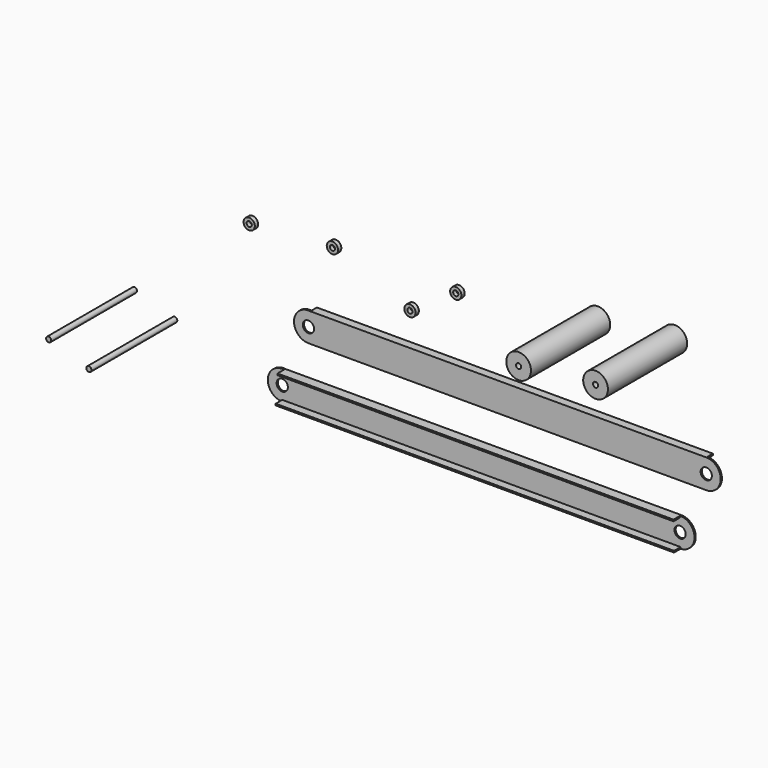
from build123d import *

# Parameters (mm, degrees)
F1_DEPTH  = 4.7752
F2_D      = 34.671
F2_DEPTH  = 4.7752
F2_TIP    = 10.4162192612
F4_DEPTH  = 25.4
F6_DEPTH  = 4.7752
F7_D      = 34.671
F7_DEPTH  = 4.7752
F7_TIP    = 10.4162192612
F9_DEPTH  = 25.4
F10_R     = 17.3355
F10_R_2   = 7.9375
F11_DEPTH = 12.7
F12_R     = 17.3355
F12_R_2   = 7.9375
F13_DEPTH = 12.7
F14_R     = 17.3355
F14_R_2   = 7.9375
F15_DEPTH = 12.7
F16_R     = 17.3355
F16_R_2   = 7.9375
F17_DEPTH = 12.7
F18_R     = 38.1
F18_R_2   = 7.9375
F19_DEPTH = 304.8
F20_R     = 38.1
F20_R_2   = 7.9375
F21_DEPTH = 304.8
F22_R     = 7.9375
F23_DEPTH = 330.2
F24_R     = 7.9375
F25_DEPTH = 330.2


# Not quite as in the source:
# - a feature names something its author has since deleted; it is built from what else it names


with BuildPart() as f1:
    # F0 (on Front) → F1 (new body)
    with BuildSketch(Plane.XZ):
        with BuildLine():
            Line((-1074.6594506346, -44.4499999817), (148.4365754055, -44.414878516))
            Line((148.4365754055, -44.414878516), (151.9724341991, -44.414776983))
            ThreePointArc((151.9724341991, -44.414776983), (194.6442914443, 0.8913507924), (150.1900805819, 44.4499980552))
            Line((150.1900805819, 44.4499980552), (-1069.0098660753, 44.0893441833))
            ThreePointArc((-1069.0098660753, 44.0893441833), (-1119.0205120843, 2.8305422757), (-1074.6594506346, -44.4499999817))
        make_face()
    extrude(amount=F1_DEPTH)

    # F2
    with Locations(Plane(origin=(0, 0, 0), x_dir=(1, 0, 0), z_dir=(0, 1, 0))):
        with Locations((-1074.6607270259, 0), (150.2032294209, 0)):
            Hole(F2_D / 2, depth=F2_DEPTH)
            with Locations((0, 0, -(F2_DEPTH + F2_TIP / 2))):  # 118° drill point
                Cone(0, F2_D / 2, F2_TIP, mode=Mode.SUBTRACT)

    # F3 (on face) → F4 (join)
    with BuildSketch(Plane.XZ.offset(4.7752)):
        Polygon((-1074.6595877555, -39.6747999836), (-1074.6594506346, -44.4499999817), (151.9724341991, -44.414776983), (151.9722970782, -39.639576985), align=None)
        Polygon((150.1900805819, 44.4499980552), (-1069.0098660753, 44.0893441833), (-1069.0084535143, 39.3141446012), (150.1900805819, 39.6747980552), align=None)
    extrude(amount=F4_DEPTH)


with BuildPart() as f6:
    # F5 (on Front) → F6 (new body)
    with BuildSketch(Plane.XZ):
        with BuildLine():
            Line((-994.0826163973, 139.9620227242), (229.0134096428, 139.9971441899))
            Line((229.0134096428, 139.9971441899), (232.5492684364, 139.9972457228))
            ThreePointArc((232.5492684364, 139.9972457228), (275.2211256816, 185.3033734983), (230.7669148192, 228.8620207611))
            Line((230.7669148192, 228.8620207611), (-988.433031838, 228.5013668892))
            ThreePointArc((-988.433031838, 228.5013668892), (-1038.443677847, 187.2425649815), (-994.0826163973, 139.9620227242))
        make_face()
    extrude(amount=F6_DEPTH)

    # F7
    with Locations(Plane(origin=(0, 0, 0), x_dir=(1, 0, 0), z_dir=(0, 1, 0))):
        with Locations((-994.0838927886, -184.4120227059), (230.7800636583, -184.4120227059)):
            Hole(F7_D / 2, depth=F7_DEPTH)
            with Locations((0, 0, -(F7_DEPTH + F7_TIP / 2))):  # 118° drill point
                Cone(0, F7_D / 2, F7_TIP, mode=Mode.SUBTRACT)

    # F8 (on face) → F9 (join)
    with BuildSketch(Plane.XZ.offset(4.7752)):
        Polygon((230.7669148192, 228.8620207611), (-988.433031838, 228.5013668892), (-988.431619277, 223.7261670981), (230.7669148192, 224.0868205521), align=None)
        Polygon((-994.0840289583, 144.7372225153), (-994.0826163973, 139.9620227242), (232.5492684364, 139.9972457228), (232.5492684364, 145.1000752608), align=None)
    extrude(amount=-F9_DEPTH)


with BuildPart() as f11:
    # F10 (on Front) → F11 (new body)
    with BuildSketch(Plane.XZ):
        with Locations((-675.2595901489, 335.0400328636)):
            Circle(F10_R)
        with Locations((-675.2595901489, 335.0400328636)):
            Circle(F10_R_2, mode=Mode.SUBTRACT)
    extrude(amount=F11_DEPTH)


with BuildPart() as f13:
    # F12 (on face) → F13 (new body)
    with BuildSketch(Plane(origin=(0, 0, 0), x_dir=(-1, 0, 0), z_dir=(0, 1, 0))):
        with Locations((924.1690039635, 419.3358123302)):
            Circle(F12_R)
        with Locations((924.1690039635, 419.3358123302)):
            Circle(F12_R_2, mode=Mode.SUBTRACT)
    extrude(amount=F13_DEPTH)


with BuildPart() as f15:
    # F14 (on Front) → F15 (new body)
    with BuildSketch(Plane.XZ):
        with Locations((-534.1455936432, 428.1651079655)):
            Circle(F14_R)
        with Locations((-534.1455936432, 428.1651079655)):
            Circle(F14_R_2, mode=Mode.SUBTRACT)
    extrude(amount=F15_DEPTH)


with BuildPart() as f17:
    # F16 (on Front) → F17 (new body)
    with BuildSketch(Plane.XZ):
        with Locations((-1170.1385974884, 409.0607762337)):
            Circle(F16_R)
        with Locations((-1170.1385974884, 409.0607762337)):
            Circle(F16_R_2, mode=Mode.SUBTRACT)
    extrude(amount=F17_DEPTH)


with BuildPart() as f19:
    # F18 (on Front) → F19 (new body)
    with BuildSketch(Plane.XZ):
        with Locations((-350.7515192032, 285.3947877884)):
            Circle(F18_R)
        with Locations((-350.7515192032, 285.3947877884)):
            Circle(F18_R_2, mode=Mode.SUBTRACT)
    extrude(amount=-F19_DEPTH)


with BuildPart() as f21:
    # F20 (on Front) → F21 (new body)
    with BuildSketch(Plane.XZ):
        with Locations((-113.8105988503, 311.6956949234)):
            Circle(F20_R)
        with Locations((-113.8105988503, 311.6956949234)):
            Circle(F20_R_2, mode=Mode.SUBTRACT)
    extrude(amount=-F21_DEPTH)


with BuildPart() as f23:
    # F22 (on Front) → F23 (new body)
    with BuildSketch(Plane.XZ):
        with Locations((-1409.6375703812, 67.0676827431)):
            Circle(F22_R)
    extrude(amount=F23_DEPTH)


with BuildPart() as f25:
    # F24 (on Front) → F25 (new body)
    with BuildSketch(Plane.XZ):
        with Locations((-1533.5742235184, 107.0293113589)):
            Circle(F24_R)
    extrude(amount=F25_DEPTH)


solid = Compound([f1.part, f6.part, f11.part, f13.part, f15.part, f17.part, f19.part, f21.part, f23.part, f25.part])
